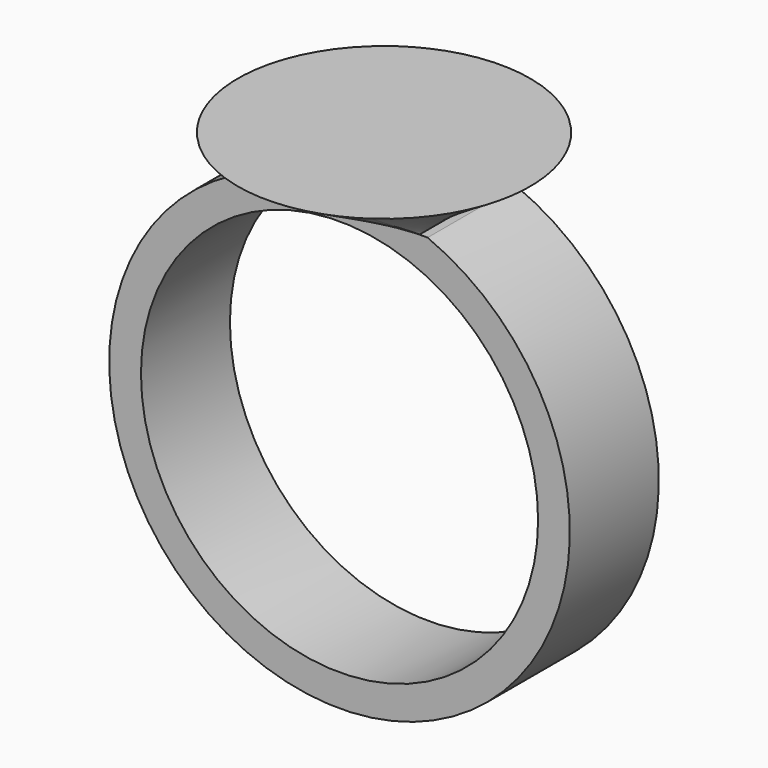
from build123d import *

# Parameters (mm, degrees)
F0_R     = 14.5
F0_R_2   = 12.5
F1_DEPTH = 7
F2_W     = 48.194617033
F2_H     = 4.0483484045
F3_DEPTH = 27.99757
F5_W     = 10.1034124382
F5_H     = 6.9993771613


# Not quite as in the source:
# - the arcs of a loft's sections are written as splines that run evenly, so that the points pair up as in the source's solid


with BuildPart() as f1:
    # F0 (on Front) → F1 (new body)
    with BuildSketch(Plane.XZ):
        Circle(F0_R)
        Circle(F0_R_2, mode=Mode.SUBTRACT)
    extrude(amount=F1_DEPTH)

    # F2 (on Front) → F3 (cut)
    with BuildSketch(Plane.XZ):
        with Locations((7.1328040212, 15.4222766869)):
            Rectangle(F2_W, F2_H)
    extrude(amount=F3_DEPTH, mode=Mode.SUBTRACT)


with BuildPart() as f8:
    # F7 (on offset) → F8 section 0
    with BuildSketch(Plane.XY.offset(16)):
        with BuildLine():
            add(Edge.make_bspline(
                [(7.565968402, 1.7430809523), (6.880091644, 2.7334639001), (5.9975628433, 3.5870814841), (3.9722215545, 4.89212321), (2.8302059518, 5.3430338738), (0.4596167417, 5.7736706573), (-0.76802414, 5.7532273399), (-3.1229605537, 5.2438986345), (-4.2493295187, 4.7552136457), (-5.2397124665, 4.0693368877)],
                knots=[0, 0, 0, 0, 0.25, 0.25, 0.5, 0.5, 0.75, 0.75, 1, 1, 1, 1], degree=3))
            add(Edge.make_bspline(
                [(-5.2397124665, 4.0693368877), (-6.2300954144, 3.3834601297), (-7.0837129984, 2.500931329), (-8.3887547243, 0.4755900402), (-8.8396653881, -0.6664255625), (-9.2703021716, -3.0370147726), (-9.2498588542, -4.2646556543), (-8.7405301488, -6.619592068), (-8.25184516, -7.745961033), (-7.565968402, -8.7363439808)],
                knots=[0, 0, 0, 0, 0.25, 0.25, 0.5, 0.5, 0.75, 0.75, 1, 1, 1, 1], degree=3))
            add(Edge.make_bspline(
                [(-7.565968402, -8.7363439808), (-6.880091644, -9.7267269287), (-5.9975628433, -10.5803445126), (-3.9722215545, -11.8853862386), (-2.8302059518, -12.3362969023), (-0.4596167417, -12.7669336859), (0.76802414, -12.7464903685), (3.1229605537, -12.2371616631), (4.2493295187, -11.7484766742), (5.2397124665, -11.0625999162)],
                knots=[0, 0, 0, 0, 0.25, 0.25, 0.5, 0.5, 0.75, 0.75, 1, 1, 1, 1], degree=3))
            add(Edge.make_bspline(
                [(5.2397124665, -11.0625999162), (6.2300954144, -10.3767231583), (7.0837129984, -9.4941943576), (8.3887547243, -7.4688530688), (8.8396653881, -6.326837466), (9.2703021716, -3.9562482559), (9.2498588542, -2.7286073742), (8.7405301488, -0.3736709606), (8.25184516, 0.7526980044), (7.565968402, 1.7430809523)],
                knots=[0, 0, 0, 0, 0.25, 0.25, 0.5, 0.5, 0.75, 0.75, 1, 1, 1, 1], degree=3))
        make_face()
    # F5 (on offset) → F8 section 1
    with BuildSketch(Plane.XY.offset(13.41)):
        with Locations((-0.0026880298, -3.4996885806)):
            Rectangle(F5_W, F5_H)
    loft(ruled=True)


solid = Compound([f1.part, f8.part])
